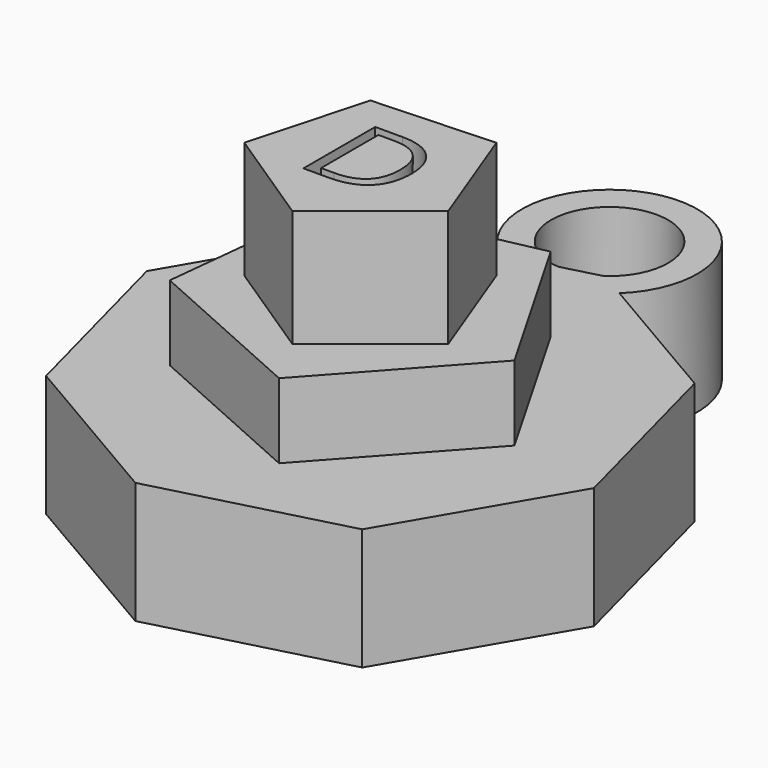
from build123d import *

# Parameters (mm, degrees)
F1_DEPTH     = 6.604
F3_DEPTH     = 10.668
F5_DEPTH     = 6.35
F6_TEXT_SIZE = 6.8207940791
F7_DEPTH     = 6.35
F8_R         = 4.7625
F8_R_2       = 3.175
F9_DEPTH     = 6.604


# Not quite as in the source:
# - Text() gives the source's letters only with a copy of the font that has no kerning and outlines rounded to 1/6400 em; it was checked with that copy


with BuildPart() as f1:
    # F0 (on Top) → F1 (new body)
    with BuildSketch(Plane.XY):
        Polygon((8.3164526498, -10.9453005611), (13.620116313, -1.8588761848), (10.9453005611, 8.3164526498), (1.8588761848, 13.620116313), (-8.3164526498, 10.9453005611), (-13.620116313, 1.8588761848), (-10.9453005611, -8.3164526498), (-1.8588761848, -13.620116313), align=None)
    extrude(amount=F1_DEPTH)

    # F2 (on Top) → F3 (join)
    with BuildSketch(Plane.XY):
        Polygon((8.5510347221, -0.9116810715), (3.5094752725, 7.850792349), (-6.3820597211, 5.7637375818), (-7.4538050983, -4.2886066212), (1.7753548248, -8.4142422381), align=None)
    extrude(amount=F3_DEPTH)

    # F4 (on face) → F5 (join)
    with BuildSketch(Plane.XY.offset(10.668)):
        Polygon((5.4153916511, -1.4885658697), (3.0891583217, 4.690351367), (-3.5061868116, 4.3873624337), (-5.2561009422, -1.9788122621), (0.2577377811, -5.610335669), align=None)
    extrude(amount=F5_DEPTH)

    # F6 (on face) → F7 (cut)
    with BuildSketch(Plane.XY.offset(17.018)):
        with Locations((-2.4991815805, -2.2528233756)):
            Text('D', F6_TEXT_SIZE, font='Open Sans', text_align=(TextAlign.LEFT, TextAlign.BOTTOM))
    extrude(amount=-F7_DEPTH, mode=Mode.SUBTRACT)

    # F8 (on Top) → F9 (join, through all)
    with BuildSketch(Plane.XY):
        with Locations((0, 16.2293631583)):
            Circle(F8_R)
        with Locations((0, 16.2293631583)):
            Circle(F8_R_2, mode=Mode.SUBTRACT)
    extrude(amount=F9_DEPTH)


solid = f1.part
